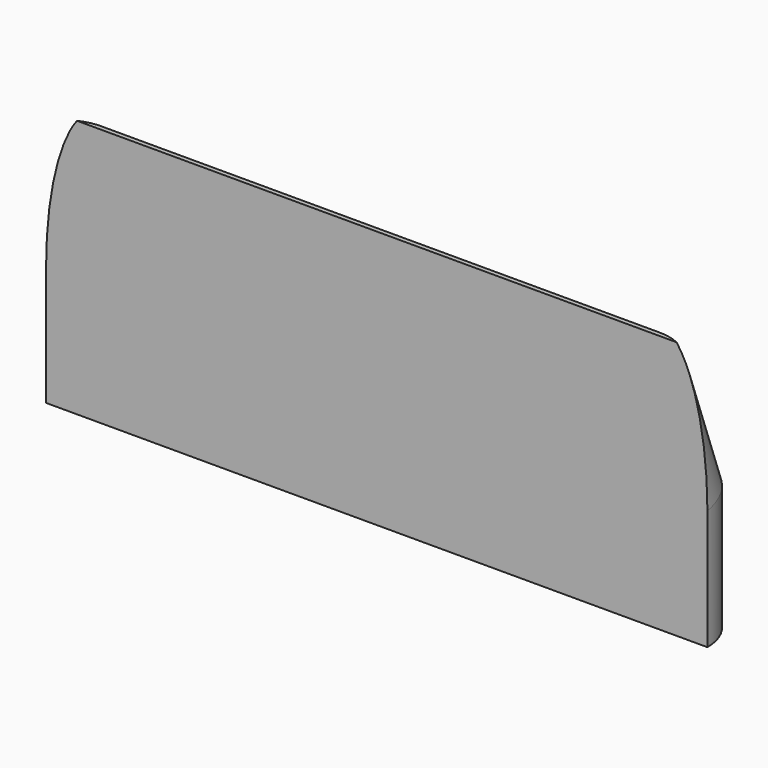
from build123d import *

# Parameters (mm, degrees)
F0_W     = 65.000124
F0_H     = 5.08
F1_DEPTH = 25.4
F2_SIZE2 = 4.6224219752
F2_SIZE  = 12.7
F3_R     = 5.07999


# Not quite as in the source:
# - a fillet or chamfer is up to 0.001 mm smaller than in the source, because OpenCascade refuses the exact size


with BuildPart() as f1:
    # F0 (on Top) → F1 (new body)
    with BuildSketch(Plane.XY):
        with Locations((-11.0949875303, 2.54)):
            Rectangle(F0_W, F0_H)
    extrude(amount=F1_DEPTH)

    # F2
    f2_edges = [f1.edges().sort_by_distance(p)[0] for p in [
        (-11.094988, 5.08, 25.4),
    ]]
    f2_side = f1.faces().sort_by_distance((-11.094988, 5.08, 12.7))[0]
    chamfer(f2_edges, length=F2_SIZE, length2=F2_SIZE2, reference=f2_side)

    # F3 (radius 5.08 in the source; OpenCascade refuses exactly that, so slightly less here)
    f3_edges = [f1.edges().sort_by_distance(p)[0] for p in [
        (21.405074, 2.768789, 19.05),
        (21.405074, 5.08, 6.35),
        (-43.59505, 5.08, 6.35),
        (-43.59505, 2.768789, 19.05),
    ]]
    fillet(f3_edges, radius=F3_R)


solid = f1.part
